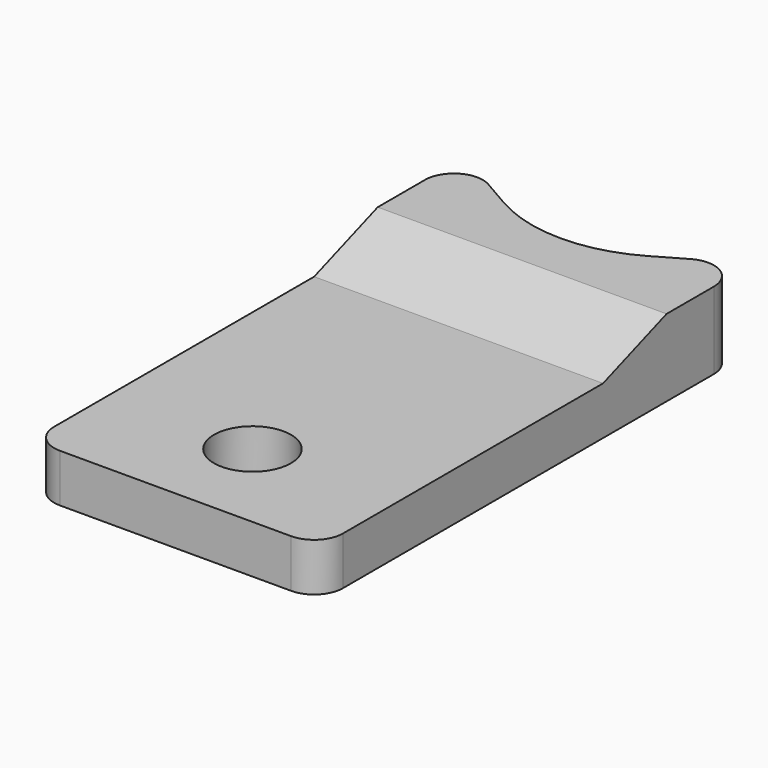
from build123d import *

# Parameters (mm, degrees)
F0_R     = 4
F0_W     = 8
F0_H     = 19
F1_DEPTH = 5
F0_H_2   = 1
F2_DEPTH = 8
F3_DEPTH = 5
F4_R     = 3
F5_SIZE2 = 2.99999
F5_SIZE  = 8.242422


# Not quite as in the source:
# - a fillet or chamfer is up to 0.001 mm smaller than in the source, because OpenCascade refuses the exact size


with BuildPart() as f1:
    # F0 (on Top) → F1 (new body)
    with BuildSketch(Plane.XY):
        Polygon((-15, 20), (-15, -25), (15, -25), (15, 20), (4, 20), (4, 1), (-4, 1), (-4, 20), align=None)
        with Locations((0, -15)):
            Circle(F0_R, mode=Mode.SUBTRACT)
        with Locations((0, 10.5)):
            Rectangle(F0_W, F0_H)
        with BuildLine():
            Line((-15, 25), (-15, 20))
            Line((-15, 20), (-4, 20))
            Line((-4, 20), (-4, 21))
            Line((-4, 21), (4, 21))
            Line((4, 21), (4, 20))
            Line((4, 20), (15, 20))
            Line((15, 20), (15, 25))
            Line((15, 25), (15, 31.3397459622))
            Line((15, 31.3397459622), (7.5, 27.0096189432))
            ThreePointArc((7.5, 27.0096189432), (0, 25), (-7.5, 27.0096189432))
            Line((-7.5, 27.0096189432), (-15, 31.3397459622))
            Line((-15, 31.3397459622), (-15, 25))
        make_face()
    extrude(amount=F1_DEPTH)

    # F0 (on Top) → F2 (join)
    with BuildSketch(Plane.XY):
        with Locations((0, 20.5)):
            Rectangle(F0_W, F0_H_2)
        with BuildLine():
            Line((-15, 25), (-15, 20))
            Line((-15, 20), (-4, 20))
            Line((-4, 20), (-4, 21))
            Line((-4, 21), (4, 21))
            Line((4, 21), (4, 20))
            Line((4, 20), (15, 20))
            Line((15, 20), (15, 25))
            Line((15, 25), (15, 31.3397459622))
            Line((15, 31.3397459622), (7.5, 27.0096189432))
            ThreePointArc((7.5, 27.0096189432), (0, 25), (-7.5, 27.0096189432))
            Line((-7.5, 27.0096189432), (-15, 31.3397459622))
            Line((-15, 31.3397459622), (-15, 25))
        make_face()
    extrude(amount=F2_DEPTH)

    # F0 (on Top) → F3 (join)
    with BuildSketch(Plane.XY):
        with Locations((0, 10.5)):
            Rectangle(F0_W, F0_H)
    extrude(amount=-F3_DEPTH)

    # F4
    f4_edges = [f1.edges().sort_by_distance(p)[0] for p in [
        (-15, 31.339746, 4),
        (15, 31.339746, 4),
        (-15, -25, 2.5),
        (15, -25, 2.5),
    ]]
    fillet(f4_edges, radius=F4_R)

    # F5 (size 8.2424322584 and 3 in the source; OpenCascade refuses exactly that, so slightly less here)
    f5_edges = [f1.edges().sort_by_distance(p)[0] for p in [
        (0, 20, 5),
    ]]
    f5_side = f1.faces().sort_by_distance((0, -1.950066, 5))[0]
    chamfer(f5_edges, length=F5_SIZE, length2=F5_SIZE2, reference=f5_side)


solid = f1.part
